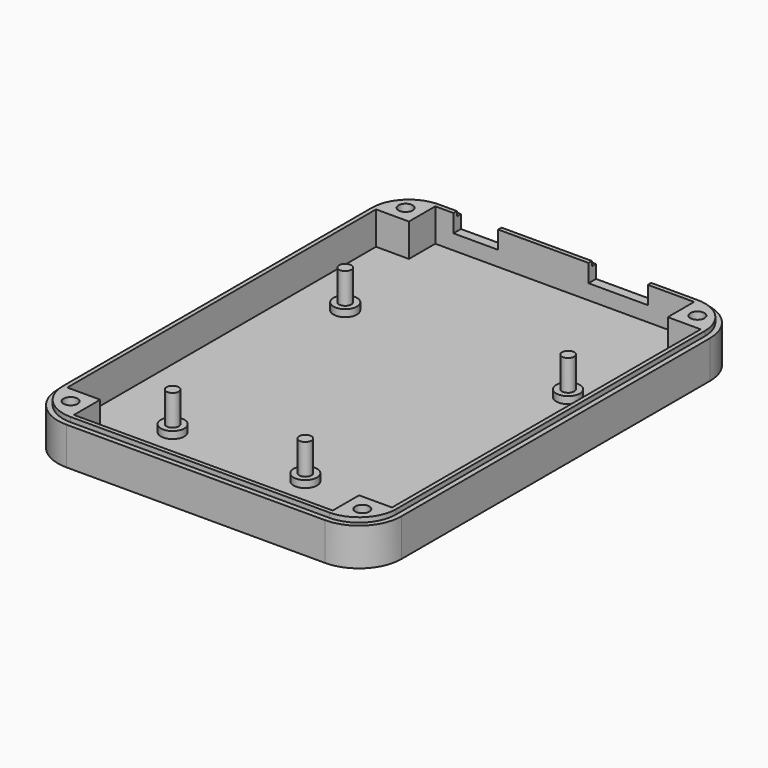
from build123d import *

# Parameters (mm, degrees)
F1_DEPTH  = 2
F2_R      = 2.5
F3_DEPTH  = 1.5
F4_R      = 1.3
F5_DEPTH  = 1.5
F7_DEPTH  = 7
F8_R      = 1.5
F9_DEPTH  = 10
F10_W     = 12.6
F10_H     = 2
F10_W_2   = 9.5
F11_DEPTH = 3.8
F12_R     = 3
F13_DEPTH = 0.4
F14_SIZE  = 1.49999
F15_W     = 19.2
F15_H     = 1.1
F16_DEPTH = 1
F17_DEPTH = 5


# Not quite as in the source:
# - a fillet or chamfer is up to 0.001 mm smaller than in the source, because OpenCascade refuses the exact size


with BuildPart() as f1:
    # F0 (on Top) → F1 (new body)
    with BuildSketch(Plane.XY):
        with BuildLine():
            Line((27.5, 63.5), (-27.5, 63.5))
            ThreePointArc((-27.5, 63.5), (-33.8639610307, 60.8639610307), (-36.5, 54.5))
            Line((-36.5, 54.5), (-36.5, -27.5))
            ThreePointArc((-36.5, -27.5), (-33.8639610307, -33.8639610307), (-27.5, -36.5))
            Line((-27.5, -36.5), (27.5, -36.5))
            ThreePointArc((27.5, -36.5), (33.8639610307, -33.8639610307), (36.5, -27.5))
            Line((36.5, -27.5), (36.5, 54.5))
            ThreePointArc((36.5, 54.5), (33.8639610307, 60.8639610307), (27.5, 63.5))
        make_face()
    extrude(amount=F1_DEPTH)

    # F2 (on face) → F3 (join)
    with BuildSketch(Plane.XY.offset(2)):
        with Locations((-19.24, -18.6)):
            Circle(F2_R)
        with Locations((8.96, -18.6)):
            Circle(F2_R)
        with Locations((24.16, 32.2)):
            Circle(F2_R)
        with Locations((-24.24, 33.5)):
            Circle(F2_R)
    extrude(amount=F3_DEPTH)

    # F4 (on face) → F5 (join)
    with BuildSketch(Plane.XY.offset(3.5)):
        with Locations((-19.24, -18.6)):
            Circle(F4_R)
        with Locations((8.96, -18.6)):
            Circle(F4_R)
        with Locations((24.16, 32.2)):
            Circle(F4_R)
        with Locations((-24.24, 33.5)):
            Circle(F4_R)
    extrude(amount=F5_DEPTH)

    # F6 (on face) → F7 (join)
    with BuildSketch(Plane.XY.offset(2)):
        with BuildLine():
            Line((27.5, 63.5), (-27.5, 63.5))
            ThreePointArc((-27.5, 63.5), (-33.8639610307, 60.8639610307), (-36.5, 54.5))
            Line((-36.5, 54.5), (-36.5, -27.5))
            ThreePointArc((-36.5, -27.5), (-33.8639610307, -33.8639610307), (-27.5, -36.5))
            Line((-27.5, -36.5), (27.5, -36.5))
            ThreePointArc((27.5, -36.5), (33.8639610307, -33.8639610307), (36.5, -27.5))
            Line((36.5, -27.5), (36.5, 54.5))
            ThreePointArc((36.5, 54.5), (33.8639610307, 60.8639610307), (27.5, 63.5))
        make_face()
        Polygon((-27.5, 54.5), (-27.5, 61.5), (27.5, 61.5), (27.5, 54.5), (34.5, 54.5), (34.5, -27.5), (27.5, -27.5), (27.5, -34.5), (-27.5, -34.5), (-27.5, -27.5), (-34.5, -27.5), (-34.5, 54.5), align=None, mode=Mode.SUBTRACT)
    extrude(amount=F7_DEPTH)

    # F8 (on face) → F9 (cut)
    with BuildSketch(Plane.XY.offset(9)):
        with Locations((-31, 58)):
            Circle(F8_R)
        with Locations((31, 58)):
            Circle(F8_R)
        with Locations((-31, -31)):
            Circle(F8_R)
        with Locations((31, -31)):
            Circle(F8_R)
    extrude(amount=-F9_DEPTH, mode=Mode.SUBTRACT)

    # F10 (on face) → F11 (cut)
    with BuildSketch(Plane.XY.offset(9)):
        with Locations((11.36, 62.5)):
            Rectangle(F10_W, F10_H)
        with Locations((-18.89, 62.5)):
            Rectangle(F10_W_2, F10_H)
    extrude(amount=-F11_DEPTH, mode=Mode.SUBTRACT)

    # F12 (on face) → F13 (cut)
    with BuildSketch(Plane(origin=(0, 0, 0), x_dir=(1, 0, 0), z_dir=(0, 0, -1))):
        with Locations((31, -58)):
            Circle(F12_R)
        with Locations((-31, -58)):
            Circle(F12_R)
        with Locations((-31, 31)):
            Circle(F12_R)
        with Locations((31, 31)):
            Circle(F12_R)
    extrude(amount=-F13_DEPTH, mode=Mode.SUBTRACT)

    # F14 (size 1.5 in the source; OpenCascade refuses exactly that, so slightly less here)
    f14_edges = [f1.edges().sort_by_distance(p)[0] for p in [
        (29.5, 58, 0.4),
        (-32.5, 58, 0.4),
        (29.5, -31, 0.4),
        (-32.5, -31, 0.4),
    ]]
    chamfer(f14_edges, length=F14_SIZE)

    # F15 (on face) → F16 (cut)
    with BuildSketch(Plane.XY.offset(9)):
        with BuildLine():
            Line((-23.64, 63.5), (-27.5, 63.5))
            ThreePointArc((-27.5, 63.5), (-33.8639610307, 60.8639610307), (-36.5, 54.5))
            Line((-36.5, 54.5), (-36.5, -27.5))
            ThreePointArc((-36.5, -27.5), (-33.8639610307, -33.8639610307), (-27.5, -36.5))
            Line((-27.5, -36.5), (27.5, -36.5))
            ThreePointArc((27.5, -36.5), (33.8639610307, -33.8639610307), (36.5, -27.5))
            Line((36.5, -27.5), (36.5, 54.5))
            ThreePointArc((36.5, 54.5), (33.8639610307, 60.8639610307), (27.5, 63.5))
            Line((27.5, 63.5), (17.66, 63.5))
            Line((17.66, 63.5), (17.66, 62.4))
            Line((17.66, 62.4), (27.5, 62.4))
            ThreePointArc((27.5, 62.4), (33.0861435714, 60.0861435714), (35.4, 54.5))
            Line((35.4, 54.5), (35.4, -27.5))
            ThreePointArc((35.4, -27.5), (33.0861435714, -33.0861435714), (27.5, -35.4))
            Line((27.5, -35.4), (-27.5, -35.4))
            ThreePointArc((-27.5, -35.4), (-33.0861435714, -33.0861435714), (-35.4, -27.5))
            Line((-35.4, -27.5), (-35.4, 54.5))
            ThreePointArc((-35.4, 54.5), (-33.0861435714, 60.0861435714), (-27.5, 62.4))
            Line((-27.5, 62.4), (-23.64, 62.4))
            Line((-23.64, 62.4), (-23.64, 63.5))
        make_face()
        with Locations((-4.54, 62.95)):
            Rectangle(F15_W, F15_H)
    extrude(amount=-F16_DEPTH, mode=Mode.SUBTRACT)

    # F17 (add): faces of the model
    f17_faces = [f1.faces().sort_by_distance(p)[0] for p in [
        (-19.24, -18.6, 5),
        (8.96, -18.6, 5),
        (24.16, 32.2, 5),
        (-24.24, 33.5, 5),
    ]]
    extrude(f17_faces, amount=F17_DEPTH)


solid = f1.part
